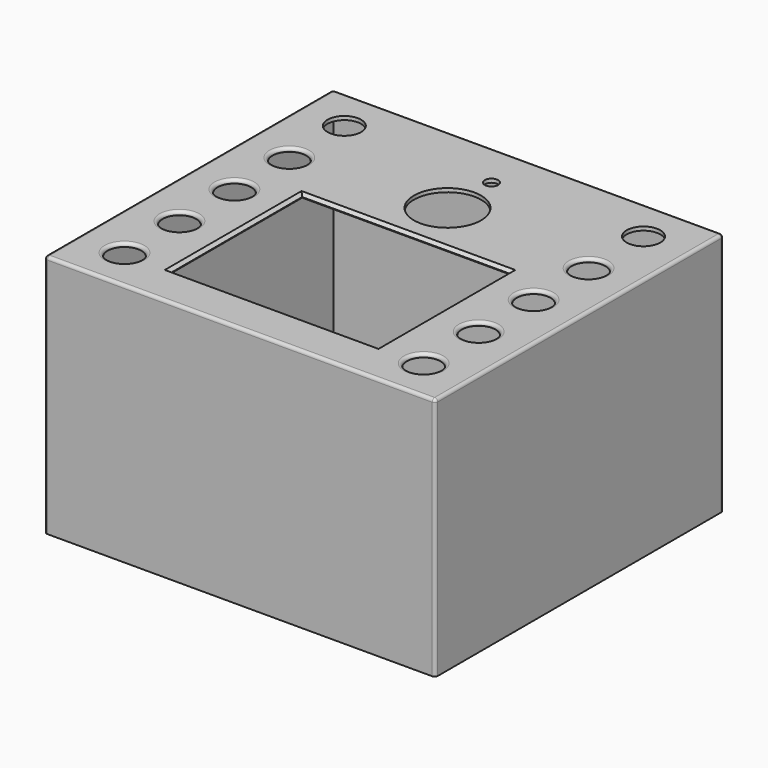
from build123d import *

# Parameters (mm, degrees)
F0_W     = 640
F0_H     = 590
F0_W_2   = 628
F0_H_2   = 578
F1_DEPTH = 400
F0_R     = 27.5
F0_W_3   = 340
F0_H_3   = 270
F0_R_2   = 55
F0_R_3   = 11
F2_DEPTH = 6
F3_R     = 5
F4_SIZE  = 5


# Not quite as in the source:
# - a feature names something its author has since deleted; it is built from what else it names


with BuildPart() as f1:
    # F0 (on Top) → F1 (new body)
    with BuildSketch(Plane.XY):
        Rectangle(F0_W, F0_H)
        Rectangle(F0_W_2, F0_H_2, mode=Mode.SUBTRACT)
    extrude(amount=-F1_DEPTH)

    # F0 (on Top) → F2 (join)
    with BuildSketch(Plane.XY):
        Rectangle(F0_W_2, F0_H_2)
        with Locations((-245, -225)):
            Circle(F0_R, mode=Mode.SUBTRACT)
        with Locations((-245, -112.5)):
            Circle(F0_R, mode=Mode.SUBTRACT)
        with Locations((245, -225)):
            Circle(F0_R, mode=Mode.SUBTRACT)
        with Locations((0, -90)):
            Rectangle(F0_W_3, F0_H_3, mode=Mode.SUBTRACT)
        with Locations((245, -112.5)):
            Circle(F0_R, mode=Mode.SUBTRACT)
        with Locations((-245, 0)):
            Circle(F0_R, mode=Mode.SUBTRACT)
        with Locations((-245, 112.5)):
            Circle(F0_R, mode=Mode.SUBTRACT)
        with Locations((-245, 225)):
            Circle(F0_R, mode=Mode.SUBTRACT)
        with Locations((0, 130)):
            Circle(F0_R_2, mode=Mode.SUBTRACT)
        with Locations((245, 0)):
            Circle(F0_R, mode=Mode.SUBTRACT)
        with Locations((245, 112.5)):
            Circle(F0_R, mode=Mode.SUBTRACT)
        with Locations((0, 220)):
            Circle(F0_R_3, mode=Mode.SUBTRACT)
        with Locations((245, 225)):
            Circle(F0_R, mode=Mode.SUBTRACT)
    extrude(amount=-F2_DEPTH)

    # F3
    f3_edges = [f1.edges().sort_by_distance(p)[0] for p in [
        (0, 295, 0),
        (320, 0, 0),
        (320, 295, -200),
        (-320, 295, -200),
        (-320, 0, 0),
        (-320, -295, -200),
        (0, -295, 0),
        (320, -295, -200),
        (-272.5, 112.5, 0),
        (-272.5, 0, 0),
        (-272.5, -112.5, 0),
        (217.5, -225, 0),
        (217.5, -112.5, 0),
        (-272.5, -225, 0),
        (217.5, 0, 0),
        (217.5, 112.5, 0),
    ]]
    fillet(f3_edges, radius=F3_R)

    # F4
    f4_edges = [f1.edges().sort_by_distance(p)[0] for p in [
        (-170, -90, 0),
        (0, 45, 0),
        (170, -90, 0),
        (0, -225, 0),
    ]]
    chamfer(f4_edges, length=F4_SIZE)


solid = f1.part
